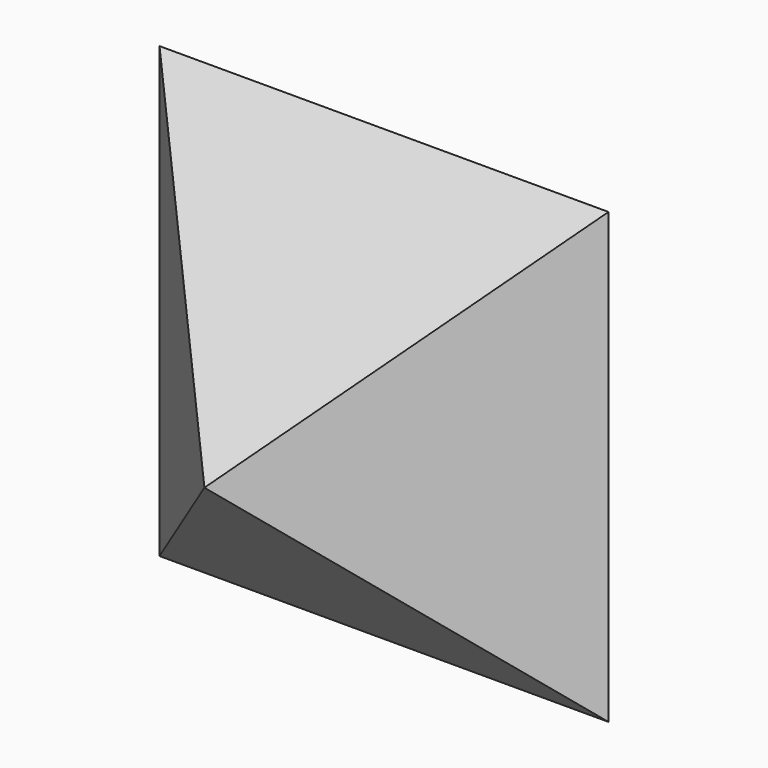
from build123d import *

# Parameters (mm, degrees)
F0_W = 127
F0_H = 127


# Not quite as in the source:
# - an extrude whose draft closes it to a point is written as a loft to that point


with BuildPart() as f1:
    # F0 (on Front) → F1 section 0
    with BuildSketch(Plane.XZ, mode=Mode.PRIVATE) as f1_s0:
        Rectangle(F0_W, F0_H)
    loft([f1_s0.sketch, Vertex(0, -63.5, 0)], ruled=True)


solid = f1.part
